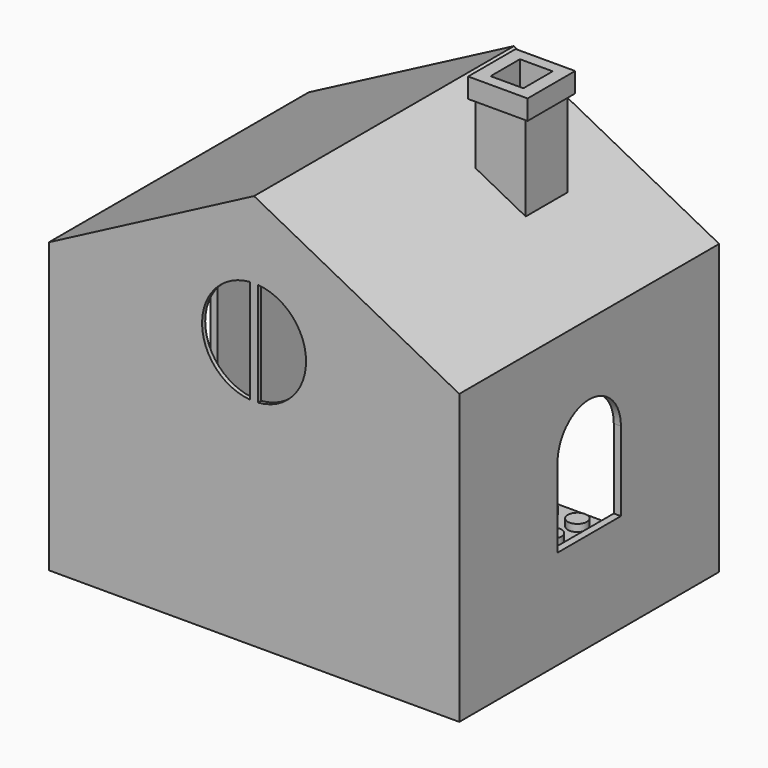
from build123d import *

# Parameters (mm, degrees)
F1_DEPTH  = 41
F3_DEPTH  = 25
F5_DEPTH  = 25
F7_DEPTH  = 41
F8_DEPTH  = 40
F10_R     = 2.4
F11_DEPTH = 1.8
F12_DEPTH = 25
F14_W     = 12.6157701015
F14_H     = 13.207135722
F14_W_2   = 8.2791037858
F14_H_2   = 9.2647057027
F14_W_3   = 15.008058399
F14_H_3   = 15.008058399
F16_DEPTH = 5


# Not quite as in the source:
# - a feature names something its author has since deleted; it is built from what else it names


with BuildPart() as f1:
    # F0 (on Front) → F1 (new body, symmetric)
    with BuildSketch(Plane.XZ):
        Polygon((-51.8000006676, -1.8000006676), (0, -1.8000006676), (51.8000006676, -1.8000006676), (51.8000006676, 71.0895588475), (0, 98.1999993324), (-51.8000006676, 71.0895588475), align=None)
        Polygon((50, 0), (0, 0), (-50, 0), (-50, 70), (0, 96.1683785092), (50, 70), align=None, mode=Mode.SUBTRACT)
        Polygon((-50, 0), (0, 0), (50, 0), (50, 70), (0, 96.1683785092), (-50, 70), align=None)
    extrude(amount=F1_DEPTH, both=True)

    # F2 (on face) → F3 (cut)
    with BuildSketch(Plane(origin=(-51.8000006676, 0, 0), x_dir=(0, -1, 0), z_dir=(-1, 0, 0))):
        with BuildLine():
            Line((-10, 43.1999993324), (-10, 23.1999993324))
            Line((-10, 23.1999993324), (10, 23.1999993324))
            Line((10, 23.1999993324), (10, 43.1999993324))
            ThreePointArc((10, 43.1999993324), (0, 53.1999993324), (-10, 43.1999993324))
        make_face()
    extrude(amount=-F3_DEPTH, mode=Mode.SUBTRACT)

    # F4 (on face) → F5 (cut)
    with BuildSketch(Plane.YZ.offset(51.8000006676)):
        with BuildLine():
            Line((-10, 43.1999993324), (-10, 23.1999993324))
            Line((-10, 23.1999993324), (10, 23.1999993324))
            Line((10, 23.1999993324), (10, 43.1999993324))
            ThreePointArc((10, 43.1999993324), (0, 53.1999993324), (-10, 43.1999993324))
        make_face()
    extrude(amount=-F5_DEPTH, mode=Mode.SUBTRACT)

    # F0 (on Front) → F7 (cut)
    with BuildSketch(Plane.XZ):
        Polygon((-50, 0), (0, 0), (50, 0), (50, 70), (0, 96.1683785092), (-50, 70), align=None)
    extrude(amount=-F7_DEPTH, mode=Mode.SUBTRACT)

    # F0 (on Front) → F8 (cut)
    with BuildSketch(Plane.XZ):
        Polygon((-50, 0), (0, 0), (50, 0), (50, 70), (0, 96.1683785092), (-50, 70), align=None)
    extrude(amount=F8_DEPTH, mode=Mode.SUBTRACT)

    # F10 (on Top) → F11 (join)
    with BuildSketch(Plane.XY):
        with Locations((-44, 36)):
            Circle(F10_R)
        with Locations((-44, 28)):
            Circle(F10_R)
        with Locations((-44, 20)):
            Circle(F10_R)
        with Locations((-44, 12)):
            Circle(F10_R)
        with Locations((-44, 4)):
            Circle(F10_R)
        with Locations((-44, -4)):
            Circle(F10_R)
        with Locations((-44, -12)):
            Circle(F10_R)
        with Locations((-44, -20)):
            Circle(F10_R)
        with Locations((-44, -28)):
            Circle(F10_R)
        with Locations((-44, -36)):
            Circle(F10_R)
        with Locations((-36, 36)):
            Circle(F10_R)
        with Locations((-36, 28)):
            Circle(F10_R)
        with Locations((-36, 20)):
            Circle(F10_R)
        with Locations((-36, 12)):
            Circle(F10_R)
        with Locations((-36, 4)):
            Circle(F10_R)
        with Locations((-36, -4)):
            Circle(F10_R)
        with Locations((-36, -12)):
            Circle(F10_R)
        with Locations((-36, -20)):
            Circle(F10_R)
        with Locations((-36, -28)):
            Circle(F10_R)
        with Locations((-36, -36)):
            Circle(F10_R)
        with Locations((-28, 36)):
            Circle(F10_R)
        with Locations((-28, 28)):
            Circle(F10_R)
        with Locations((-28, 20)):
            Circle(F10_R)
        with Locations((-28, 12)):
            Circle(F10_R)
        with Locations((-28, 4)):
            Circle(F10_R)
        with Locations((-28, -4)):
            Circle(F10_R)
        with Locations((-28, -12)):
            Circle(F10_R)
        with Locations((-28, -20)):
            Circle(F10_R)
        with Locations((-28, -28)):
            Circle(F10_R)
        with Locations((-28, -36)):
            Circle(F10_R)
        with Locations((-20, 36)):
            Circle(F10_R)
        with Locations((-20, 28)):
            Circle(F10_R)
        with Locations((-20, 20)):
            Circle(F10_R)
        with Locations((-20, 12)):
            Circle(F10_R)
        with Locations((-20, 4)):
            Circle(F10_R)
        with Locations((-20, -4)):
            Circle(F10_R)
        with Locations((-20, -12)):
            Circle(F10_R)
        with Locations((-20, -20)):
            Circle(F10_R)
        with Locations((-20, -28)):
            Circle(F10_R)
        with Locations((-20, -36)):
            Circle(F10_R)
        with Locations((-12, 36)):
            Circle(F10_R)
        with Locations((-12, 28)):
            Circle(F10_R)
        with Locations((-12, 20)):
            Circle(F10_R)
        with Locations((-12, 12)):
            Circle(F10_R)
        with Locations((-12, 4)):
            Circle(F10_R)
        with Locations((-12, -4)):
            Circle(F10_R)
        with Locations((-12, -12)):
            Circle(F10_R)
        with Locations((-12, -20)):
            Circle(F10_R)
        with Locations((-12, -28)):
            Circle(F10_R)
        with Locations((-12, -36)):
            Circle(F10_R)
        with Locations((-4, 36)):
            Circle(F10_R)
        with Locations((-4, 28)):
            Circle(F10_R)
        with Locations((-4, 20)):
            Circle(F10_R)
        with Locations((-4, 12)):
            Circle(F10_R)
        with Locations((-4, 4)):
            Circle(F10_R)
        with Locations((-4, -4)):
            Circle(F10_R)
        with Locations((-4, -12)):
            Circle(F10_R)
        with Locations((-4, -20)):
            Circle(F10_R)
        with Locations((-4, -28)):
            Circle(F10_R)
        with Locations((-4, -36)):
            Circle(F10_R)
        with Locations((4, 36)):
            Circle(F10_R)
        with Locations((4, 28)):
            Circle(F10_R)
        with Locations((4, 20)):
            Circle(F10_R)
        with Locations((4, 12)):
            Circle(F10_R)
        with Locations((4, 4)):
            Circle(F10_R)
        with Locations((4, -4)):
            Circle(F10_R)
        with Locations((4, -12)):
            Circle(F10_R)
        with Locations((4, -20)):
            Circle(F10_R)
        with Locations((4, -28)):
            Circle(F10_R)
        with Locations((4, -36)):
            Circle(F10_R)
        with Locations((12, 36)):
            Circle(F10_R)
        with Locations((12, 28)):
            Circle(F10_R)
        with Locations((12, 20)):
            Circle(F10_R)
        with Locations((12, 12)):
            Circle(F10_R)
        with Locations((12, 4)):
            Circle(F10_R)
        with Locations((12, -4)):
            Circle(F10_R)
        with Locations((12, -12)):
            Circle(F10_R)
        with Locations((12, -20)):
            Circle(F10_R)
        with Locations((12, -28)):
            Circle(F10_R)
        with Locations((12, -36)):
            Circle(F10_R)
        with Locations((20, 36)):
            Circle(F10_R)
        with Locations((20, 28)):
            Circle(F10_R)
        with Locations((20, 20)):
            Circle(F10_R)
        with Locations((20, 12)):
            Circle(F10_R)
        with Locations((20, 4)):
            Circle(F10_R)
        with Locations((20, -4)):
            Circle(F10_R)
        with Locations((20, -12)):
            Circle(F10_R)
        with Locations((20, -20)):
            Circle(F10_R)
        with Locations((20, -28)):
            Circle(F10_R)
        with Locations((20, -36)):
            Circle(F10_R)
        with Locations((28, 36)):
            Circle(F10_R)
        with Locations((28, 28)):
            Circle(F10_R)
        with Locations((28, 20)):
            Circle(F10_R)
        with Locations((28, 12)):
            Circle(F10_R)
        with Locations((28, 4)):
            Circle(F10_R)
        with Locations((28, -4)):
            Circle(F10_R)
        with Locations((28, -12)):
            Circle(F10_R)
        with Locations((28, -20)):
            Circle(F10_R)
        with Locations((28, -28)):
            Circle(F10_R)
        with Locations((28, -36)):
            Circle(F10_R)
        with Locations((36, 36)):
            Circle(F10_R)
        with Locations((36, 28)):
            Circle(F10_R)
        with Locations((36, 20)):
            Circle(F10_R)
        with Locations((36, 12)):
            Circle(F10_R)
        with Locations((36, 4)):
            Circle(F10_R)
        with Locations((36, -4)):
            Circle(F10_R)
        with Locations((36, -12)):
            Circle(F10_R)
        with Locations((36, -20)):
            Circle(F10_R)
        with Locations((36, -28)):
            Circle(F10_R)
        with Locations((36, -36)):
            Circle(F10_R)
        with Locations((44, 36)):
            Circle(F10_R)
        with Locations((44, 28)):
            Circle(F10_R)
        with Locations((44, 20)):
            Circle(F10_R)
        with Locations((44, 12)):
            Circle(F10_R)
        with Locations((44, 4)):
            Circle(F10_R)
        with Locations((44, -4)):
            Circle(F10_R)
        with Locations((44, -12)):
            Circle(F10_R)
        with Locations((44, -20)):
            Circle(F10_R)
        with Locations((44, -28)):
            Circle(F10_R)
        with Locations((44, -36)):
            Circle(F10_R)
    extrude(amount=F11_DEPTH)

    # F9 (on face) → F12 (cut)
    with BuildSketch(Plane.XZ.offset(41)):
        with BuildLine():
            Line((-1, 52.6246078838), (-1, 78.8037083518))
            ThreePointArc((-1, 78.8037083518), (-13.1276930696, 65.7141581178), (-1, 52.6246078838))
        make_face()
        with BuildLine():
            ThreePointArc((1, 52.6246078838), (9.629746061, 56.7920330273), (13.1276930696, 65.7141581178))
            ThreePointArc((13.1276930696, 65.7141581178), (9.629746061, 74.6362832082), (1, 78.8037083518))
            Line((1, 78.8037083518), (1, 52.6246078838))
        make_face()
    extrude(amount=-F12_DEPTH, mode=Mode.SUBTRACT)

    # F14 (on offset) → F15 (join, up to the next surface of F1)
    with BuildSketch(Plane.XY.offset(110)):
        with Locations((22.7182414383, 15.0305079296)):
            Rectangle(F14_W, F14_H)
        with Locations((22.7182414383, 15.0305079296)):
            Rectangle(F14_W_2, F14_H_2, mode=Mode.SUBTRACT)
    extrude(until=Until.NEXT, dir=(0, 0, -1))

    # F14 (on offset) → F16 (join)
    with BuildSketch(Plane.XY.offset(110)):
        with Locations((22.7182414383, 15.0305079296)):
            Rectangle(F14_W_3, F14_H_3)
        with Locations((22.7182414383, 15.0305079296)):
            Rectangle(F14_W, F14_H, mode=Mode.SUBTRACT)
    extrude(amount=-F16_DEPTH)


solid = f1.part
